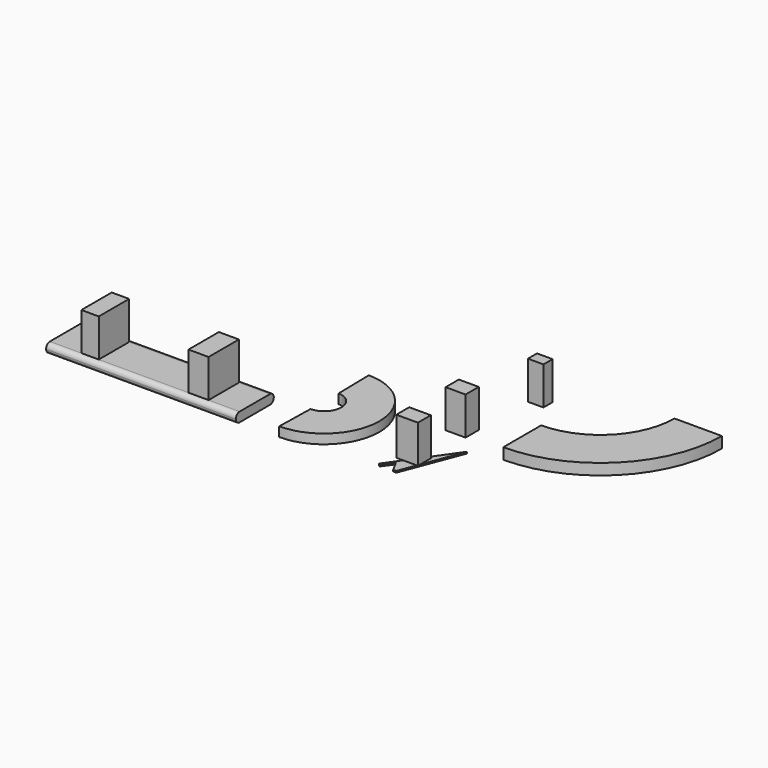
from build123d import *

# Parameters (mm, degrees)
F0_W         = 3048
F0_H         = 762
F1_DEPTH     = 152.4
F2_R         = 76.19999
F3_W         = 279.8554897308
F3_H         = 609.6
F3_W_2       = 322.9101896286
F4_DEPTH     = 609.6
F5_TEXT_SIZE = 444.2362735669
F6_DEPTH     = 25.4
F8_DEPTH     = 152.4
F9_W         = 319.8838233948
F9_H         = 265.7654285431
F10_DEPTH    = 609.6
F9_W_2       = 347.2263813019
F9_H_2       = 259.4142854214
F12_DEPTH    = 25.4
F16_DEPTH    = 177.8
F17_W        = 249.2110729218
F17_H        = 183.247089386
F18_DEPTH    = 609.6


# Not quite as in the source:
# - a fillet or chamfer is up to 0.001 mm smaller than in the source, because OpenCascade refuses the exact size
# - Text() gives the source's letters only with a copy of the font that has no kerning and outlines rounded to 1/6400 em; it was checked with that copy


with BuildPart() as f1:
    # F0 (on Top) → F1 (new body)
    with BuildSketch(Plane.XY):
        with Locations((-473.1570378005, 15.6856263056)):
            Rectangle(F0_W, F0_H)
    extrude(amount=F1_DEPTH)

    # F2 (radius 76.2 in the source; OpenCascade refuses exactly that, so slightly less here)
    f2_edges = [f1.edges().sort_by_distance(p)[0] for p in [
        (-473.157038, -365.314374, 0),
        (-473.157038, -365.314374, 152.4),
        (-473.157038, 396.685626, 0),
        (-473.157038, 396.685626, 152.4),
    ]]
    fillet(f2_edges, radius=F2_R)

    # F3 (on face) → F4 (join)
    with BuildSketch(Plane.XY.offset(152.4)):
        with Locations((-1351.541519165, 15.6856263056)):
            Rectangle(F3_W, F3_H)
        with Locations((390.5721902847, 15.6856263056)):
            Rectangle(F3_W_2, F3_H)
    extrude(amount=F4_DEPTH)

    # F5 (on face) → F6 (join)
    with BuildSketch(Plane(origin=(0, 0, 0), x_dir=(1, 0, 0), z_dir=(0, 0, -1))):
        with Locations((-1058.1827163696, -139.2217129469)):
            Text('>>>>>', F5_TEXT_SIZE, font='Open Sans', text_align=(TextAlign.LEFT, TextAlign.BOTTOM))
    extrude(amount=F6_DEPTH)


with BuildPart() as f8:
    # F7 (on face) → F8 (new body)
    with BuildSketch(Plane(origin=(0, 0, 0), x_dir=(1, 0, 0), z_dir=(0, 0, -1))):
        with BuildLine():
            ThreePointArc((1700.2901325226, -1493.442773819), (2584.098946887, -595.1095740848), (1688.4457359314, 291.4150357246))
            Line((1688.4457359314, 291.4150357246), (1701.5952358246, -320.4856263056))
            ThreePointArc((1701.5952358246, -320.4856263056), (1976.9775666616, -590.8738988833), (1711.6739044189, -871.1580634117))
            Line((1711.6739044189, -871.1580634117), (1700.2901325226, -1493.442773819))
        make_face()
    extrude(amount=-F8_DEPTH)


with BuildPart() as f10:
    # F9 (on face) → F10 (new body)
    with BuildSketch(Plane.XY.offset(152.4)):
        with Locations((3545.7324981689, 1060.8603954315)):
            Rectangle(F9_W, F9_H)
    extrude(amount=F10_DEPTH)


with BuildPart() as f10b:
    # F9 (on face) → F10, piece 2 (new body)
    with BuildSketch(Plane.XY.offset(152.4)):
        with Locations((3543.3522462845, 87.5711739063)):
            Rectangle(F9_W_2, F9_H_2)
    extrude(amount=F10_DEPTH)


with BuildPart() as f12:
    # F11 (on face) → F12 (new body)
    with BuildSketch(Plane(origin=(0, 0, 0), x_dir=(1, 0, 0), z_dir=(0, 0, -1))):
        Polygon((3141.6683739164, 90.604589339), (3116.1460778242, 72.4467462203), (3777.7855396271, -871.1580634117), (3576.3362774806, -344.5017359948), (3522.3276615143, -299.6778190136), (3548.0987528304, -270.6793210149), (3409.9054503344, 90.604589339), (3358.5171601301, 90.604589339), (3265.0129696852, -82.7660733559), align=None)
        Polygon((3522.3276615143, -299.6778190136), (3576.3362774806, -344.5017359948), (3548.0987528304, -270.6793210149), align=None)
    extrude(amount=F12_DEPTH)


with BuildPart() as f13_1:
    # F13: copy of F8
    add(f8.part.moved(Location((0, 2133.6, 0))))


with BuildPart() as f16:
    # F15 (on face) → F16 (new body)
    with BuildSketch(Plane(origin=(0, 0, 0), x_dir=(1, 0, 0), z_dir=(0, 0, -1))):
        with BuildLine():
            Line((5457.5997340124, -2933.4714412689), (6219.5997340124, -2933.4714412689))
            ThreePointArc((6219.5997340124, -2933.4714412689), (5648.0765922719, -1553.6925212688), (4268.2976722717, -982.1693795282))
            Line((4268.2976722717, -982.1693795282), (4268.2976722717, -1744.1693795282))
            ThreePointArc((4268.2976722717, -1744.1693795282), (5109.2612250077, -2092.5078885329), (5457.5997340124, -2933.4714412689))
        make_face()
    extrude(amount=-F16_DEPTH)


with BuildPart() as f18:
    # F17 (on face) → F18 (new body)
    with BuildSketch(Plane.XY.offset(177.8)):
        with Locations((3863.3390665054, 2231.0862541199)):
            Rectangle(F17_W, F17_H)
    extrude(amount=F18_DEPTH)


solid = Compound([f1.part, f8.part, f10.part, f10b.part, f12.part, f16.part, f18.part])
